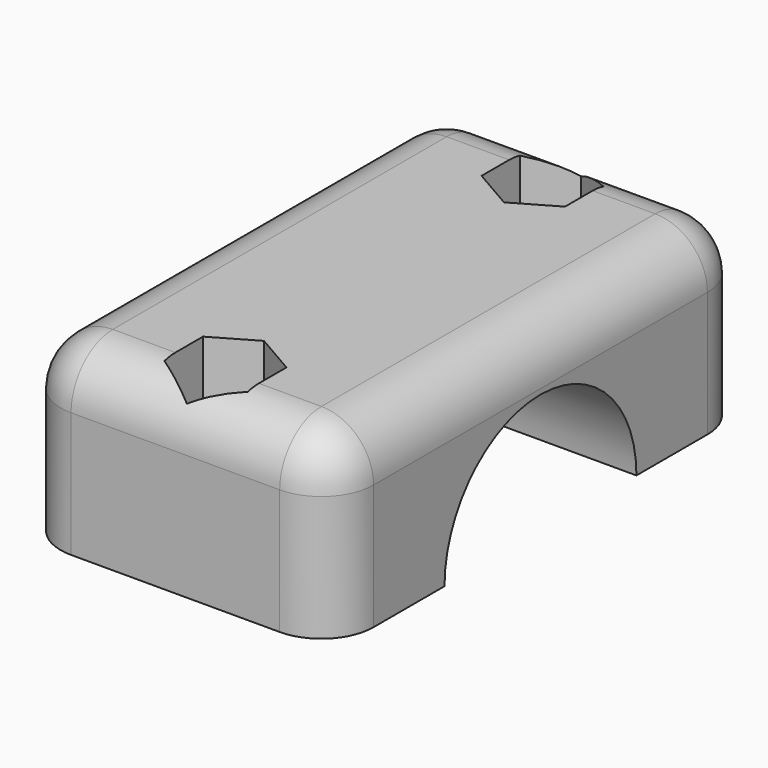
from build123d import *

# Parameters (mm, degrees)
F0_W         = 30
F0_H         = 25
F1_DEPTH     = 17
F3_DEPTH     = 50
F4_D         = 5
F5_R         = 2.5
F6_DEPTH     = 6
F7_R         = 5
F8_T1_DEPTH  = 40
F8_T3_DEPTH  = 20
F8_T6_ANGLE  = 90
F8_T8_ANGLE  = 90
F8_T10_ANGLE = 90
F8_T12_ANGLE = 90


# Not quite as in the source:
# - a fillet or chamfer that OpenCascade refuses, or shapes differently, is made with other operations: its cross-section is extruded or revolved along the edge and cut away or added


with BuildPart() as f1:
    # F0 (on Top) → F1 (new body)
    with BuildSketch(Plane.XY):
        with Locations((0, 12.5)):
            Rectangle(F0_W, F0_H)
        with Locations((0, -12.5)):
            Rectangle(F0_W, F0_H)
    extrude(amount=F1_DEPTH)

    # F2 (on face) → F3 (cut)
    with BuildSketch(Plane.YZ.offset(15)):
        with BuildLine():
            Line((-11.5, 0), (11.5, 0))
            ThreePointArc((11.5, 0), (0, 11.5), (-11.5, 0))
        make_face()
        with BuildLine():
            ThreePointArc((-11.5, 0), (0, -11.5), (11.5, 0))
            Line((11.5, 0), (-11.5, 0))
        make_face()
    extrude(amount=-F3_DEPTH, mode=Mode.SUBTRACT)

    # F4 (through all)
    with Locations(Plane(origin=(0, 0, 0), x_dir=(1, 0, 0), z_dir=(0, 0, -1))):
        with Locations((0, -19), (0, 19)):
            Hole(F4_D / 2)

    # F5 (on face) → F6 (cut)
    with BuildSketch(Plane.XY.offset(17)):
        Polygon((4, -21.3094010768), (4, -16.6905989232), (0, -14.3811978465), (-4, -16.6905989232), (-4, -21.3094010768), (0, -23.6188021535), align=None)
        with Locations((0, -19)):
            Circle(F5_R, mode=Mode.SUBTRACT)
        Polygon((4, 16.6905989232), (4, 21.3094010768), (0, 23.6188021535), (-4, 21.3094010768), (-4, 16.6905989232), (0, 14.3811978465), align=None)
        with Locations((0, 19)):
            Circle(F5_R, mode=Mode.SUBTRACT)
    extrude(amount=-F6_DEPTH, mode=Mode.SUBTRACT)

    # F7
    f7_edges = [f1.edges().sort_by_distance(p)[0] for p in [
        (-15, 25, 8.5),
        (15, 25, 8.5),
        (-15, -25, 8.5),
        (15, -25, 8.5),
    ]]
    fillet(f7_edges, radius=F7_R)

    # F8: fillet of radius 5 on 1 edges, made by hand

    # F8_s2 → F8_t1 (cut)
    with BuildSketch(Plane.XZ.offset(-20)):
        with BuildLine():
            ThreePointArc((-15, 12), (-13.5355339059, 15.5355339059), (-10, 17))
            Line((-10, 17), (-15, 17))
            Line((-15, 17), (-15, 12))
        make_face()
        with BuildLine():
            ThreePointArc((10, 17), (13.5355339059, 15.5355339059), (15, 12))
            Line((15, 12), (15, 17))
            Line((15, 17), (10, 17))
        make_face()
    extrude(amount=F8_T1_DEPTH, mode=Mode.SUBTRACT)

    # F8_s4 → F8_t3 (cut)
    with BuildSketch(Plane.YZ.offset(-10)):
        with BuildLine():
            ThreePointArc((-20, 17), (-23.5355339059, 15.5355339059), (-25, 12))
            Line((-25, 12), (-25, 17))
            Line((-25, 17), (-20, 17))
        make_face()
        with BuildLine():
            ThreePointArc((20, 17), (23.5355339059, 15.5355339059), (25, 12))
            Line((25, 12), (25, 17))
            Line((25, 17), (20, 17))
        make_face()
    extrude(amount=F8_T3_DEPTH, mode=Mode.SUBTRACT)

    # F8_s5 → F8_t6 (revolve, cut)
    with BuildSketch(Plane.XZ.offset(-20)):
        with BuildLine():
            ThreePointArc((-15, 12), (-13.5355339059, 15.5355339059), (-10, 17))
            Line((-10, 17), (-15, 17))
            Line((-15, 17), (-15, 12))
        make_face()
    revolve(axis=Axis((-10, 20, 17), (0, 0, -1)), revolution_arc=F8_T6_ANGLE, mode=Mode.SUBTRACT)

    # F8_s7 → F8_t8 (revolve, cut)
    with BuildSketch(Plane.XZ.offset(20)):
        with BuildLine():
            ThreePointArc((-10, 17), (-13.5355339059, 15.5355339059), (-15, 12))
            Line((-15, 12), (-15, 17))
            Line((-15, 17), (-10, 17))
        make_face()
    revolve(axis=Axis((-10, -20, 17), (0, 0, 1)), revolution_arc=F8_T8_ANGLE, mode=Mode.SUBTRACT)

    # F8_s9 → F8_t10 (revolve, cut)
    with BuildSketch(Plane.YZ.offset(10)):
        with BuildLine():
            ThreePointArc((-20, 17), (-23.5355339059, 15.5355339059), (-25, 12))
            Line((-25, 12), (-25, 17))
            Line((-25, 17), (-20, 17))
        make_face()
    revolve(axis=Axis((10, -20, 17), (0, 0, 1)), revolution_arc=F8_T10_ANGLE, mode=Mode.SUBTRACT)

    # F8_s11 → F8_t12 (revolve, cut)
    with BuildSketch(Plane.YZ.offset(10)):
        with BuildLine():
            ThreePointArc((20, 17), (23.5355339059, 15.5355339059), (25, 12))
            Line((25, 12), (25, 17))
            Line((25, 17), (20, 17))
        make_face()
    revolve(axis=Axis((10, 20, 17), (0, 0, -1)), revolution_arc=F8_T12_ANGLE, mode=Mode.SUBTRACT)


solid = f1.part
